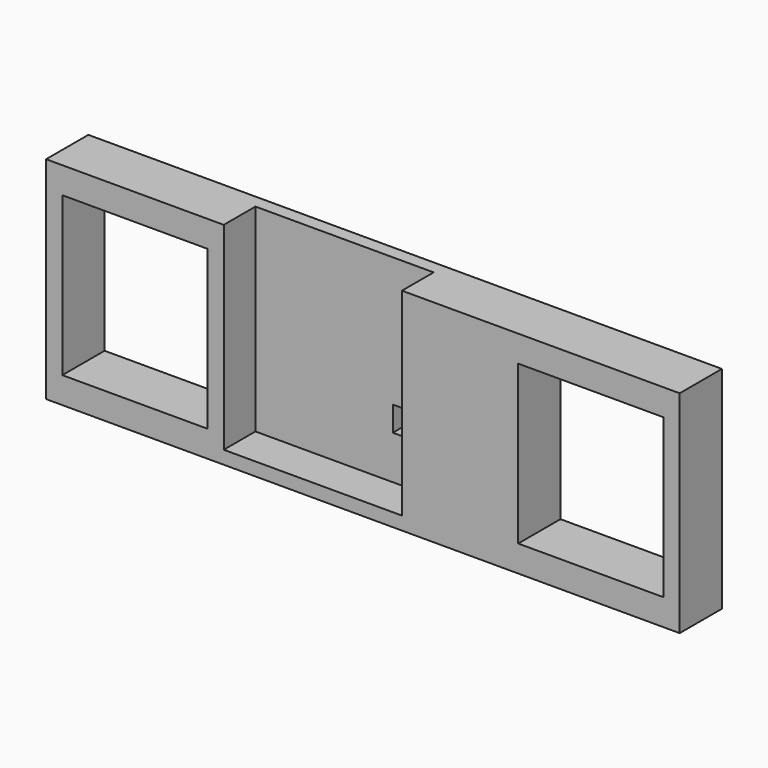
from build123d import *

# Parameters (mm, degrees)
F0_W     = 7.8232
F0_H     = 6.35
F0_W_2   = 69.85
F0_W_3   = 55.9308
F0_H_2   = 76.2
F0_W_4   = 7.7978
F0_H_3   = 12.7
F0_W_5   = 85.725
F1_DEPTH = 25.4
F0_W_6   = 16.764
F0_H_4   = 0.762
F0_H_5   = 13.4315382606
F0_W_7   = 66.0908
F0_W_8   = 2.8702
F0_H_6   = 4.9097025247
F0_H_7   = 5.1918955931
F2_DEPTH = 6.35


with BuildPart() as f1:
    # F0 (on Front) → F1 (new body)
    with BuildSketch(Plane.XZ):
        with Locations((148.4884, 56.2362195122)):
            Rectangle(F0_W, F0_H)
        with Locations((109.6518, 56.2362195122)):
            Rectangle(F0_W_2, F0_H)
        with Locations((148.4884, 49.8862195122)):
            Rectangle(F0_W, F0_H)
        with Locations((46.7614, 56.2362195122)):
            Rectangle(F0_W_3, F0_H)
        with Locations((109.6518, 49.8862195122)):
            Rectangle(F0_W_2, F0_H)
        with Locations((148.4884, 8.6112195122)):
            Rectangle(F0_W, F0_H_2)
        with Locations((46.7614, 49.8862195122)):
            Rectangle(F0_W_3, F0_H)
        with Locations((148.4884, -32.6637804878)):
            Rectangle(F0_W, F0_H)
        with Locations((-70.8279, 56.2362195122)):
            Rectangle(F0_W_4, F0_H)
        Polygon((74.7268, -2.1837804878), (74.7268, 46.7112195122), (18.796, 46.7112195122), (18.796, 3.0081151053), (18.796, -2.1837804878), align=None)
        with Locations((109.6518, -32.6637804878)):
            Rectangle(F0_W_2, F0_H)
        with Locations((148.4884, -39.0137804878)):
            Rectangle(F0_W, F0_H)
        with Locations((-109.6518, 56.2362195122)):
            Rectangle(F0_W_2, F0_H)
        with Locations((-70.8279, 49.8862195122)):
            Rectangle(F0_W_4, F0_H)
        with Locations((46.7614, -8.5337804878)):
            Rectangle(F0_W_3, F0_H_3)
        with Locations((109.6518, -39.0137804878)):
            Rectangle(F0_W_2, F0_H)
        Polygon((18.796, -29.4887804878), (74.7268, -29.4887804878), (74.7268, -14.8837804878), (18.796, -14.8837804878), (18.796, -28.3153187484), align=None)
        with Locations((46.7614, -32.6637804878)):
            Rectangle(F0_W_3, F0_H)
        with Locations((-148.4884, 56.2362195122)):
            Rectangle(F0_W, F0_H)
        with Locations((-109.6518, 49.8862195122)):
            Rectangle(F0_W_2, F0_H)
        Polygon((-66.929, 2.7259220369), (-66.929, 46.7112195122), (-74.7268, 46.7112195122), (-74.7268, -2.1837804878), (-66.929, -2.1837804878), align=None)
        with Locations((46.7614, -39.0137804878)):
            Rectangle(F0_W_3, F0_H)
        with Locations((-148.4884, 49.8862195122)):
            Rectangle(F0_W, F0_H)
        with Locations((-24.0665, -39.0137804878)):
            Rectangle(F0_W_5, F0_H)
        Polygon((-74.7268, -29.4887804878), (-66.929, -29.4887804878), (-66.929, -28.3153187484), (-66.929, -14.8837804878), (-74.7268, -14.8837804878), align=None)
        with Locations((-70.8279, -32.6637804878)):
            Rectangle(F0_W_4, F0_H)
        with Locations((-148.4884, 8.6112195122)):
            Rectangle(F0_W, F0_H_2)
        with Locations((-70.8279, -8.5337804878)):
            Rectangle(F0_W_4, F0_H_3)
        with Locations((-70.8279, -39.0137804878)):
            Rectangle(F0_W_4, F0_H)
        with Locations((-109.6518, -32.6637804878)):
            Rectangle(F0_W_2, F0_H)
        with Locations((-148.4884, -32.6637804878)):
            Rectangle(F0_W, F0_H)
        with Locations((-109.6518, -39.0137804878)):
            Rectangle(F0_W_2, F0_H)
        with Locations((-148.4884, -39.0137804878)):
            Rectangle(F0_W, F0_H)
    extrude(amount=F1_DEPTH)

    # F0 (on Front) → F2 (join)
    with BuildSketch(Plane.XZ):
        with Locations((7.5438, -2.5647804878)):
            Rectangle(F0_W_6, F0_H_4)
        with Locations((7.5438, -21.5995496181)):
            Rectangle(F0_W_6, F0_H_5)
        Polygon((-66.929, -29.4887804878), (18.796, -29.4887804878), (18.796, -28.3153187484), (15.9258, -28.3153187484), (-0.8382, -28.3153187484), (-66.929, -28.3153187484), align=None)
        with Locations((-24.0665, -32.6637804878)):
            Rectangle(F0_W_5, F0_H)
        with Locations((-33.8836, -21.5995496181)):
            Rectangle(F0_W_7, F0_H_5)
        with Locations((17.3609, -21.5995496181)):
            Rectangle(F0_W_8, F0_H_5)
        Polygon((18.796, -14.8837804878), (18.796, -2.1837804878), (15.9258, -2.1837804878), (15.9258, -2.9457804878), (15.9258, -14.8837804878), align=None)
        Polygon((-0.8382, -2.1837804878), (-66.929, -2.1837804878), (-66.929, -14.8837804878), (-0.8382, -14.8837804878), (-0.8382, -2.9457804878), align=None)
        with Locations((-33.8836, 0.2710707746)):
            Rectangle(F0_W_7, F0_H_6)
        Polygon((15.9258, -2.1837804878), (15.9258, 3.0081151053), (-0.8382, 3.0081151053), (-0.8382, 2.7259220369), (-0.8382, -2.1837804878), align=None)
        with Locations((17.3609, 0.4121673088)):
            Rectangle(F0_W_8, F0_H_7)
        Polygon((18.796, 3.0081151053), (18.796, 46.7112195122), (-66.929, 46.7112195122), (-66.929, 2.7259220369), (-0.8382, 2.7259220369), (-0.8382, 3.0081151053), (15.9258, 3.0081151053), align=None)
        with Locations((-24.0665, 49.8862195122)):
            Rectangle(F0_W_5, F0_H)
        with Locations((-24.0665, 56.2362195122)):
            Rectangle(F0_W_5, F0_H)
    extrude(amount=F2_DEPTH)


solid = f1.part
